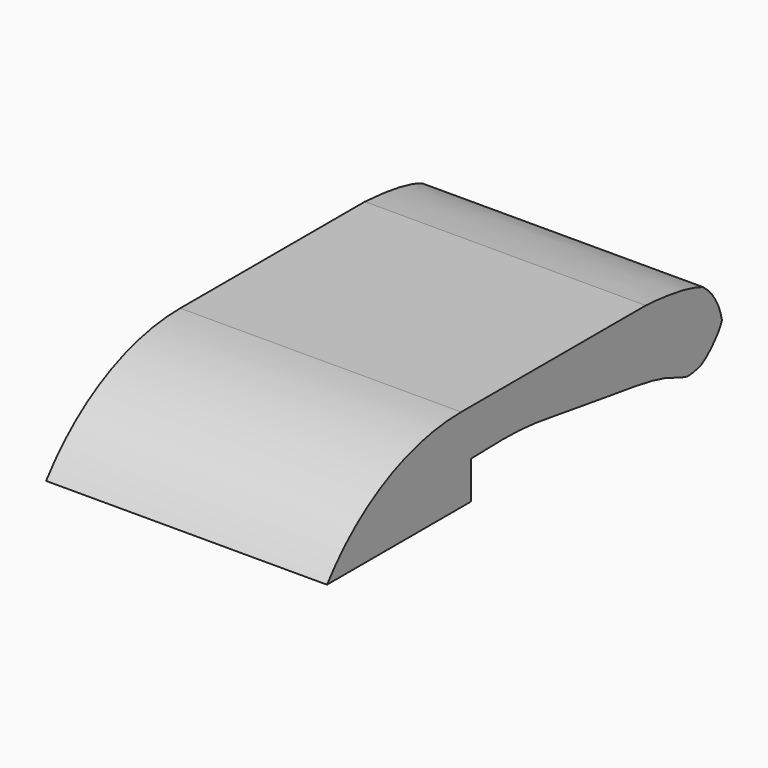
from build123d import *

# Parameters (mm, degrees)
F0_W        = 67
F0_H        = 20
F1_DEPTH    = 118
F3_T1_DEPTH = 267
F4_R        = 15
F5_T1_DEPTH = 122.9016994375
F6_DEPTH    = 67.001
F7_R        = 0.0241421356


# Not quite as in the source:
# - a fillet or chamfer that OpenCascade refuses, or shapes differently, is made with other operations: its cross-section is extruded or revolved along the edge and cut away or added


with BuildPart() as f1:
    # F0 (on Front) → F1 (new body)
    with BuildSketch(Plane.XZ):
        with Locations((6.337375957, -47.2683286667)):
            Rectangle(F0_W, F0_H)
    extrude(amount=F1_DEPTH)

    # F3: fillet of radius 50 on 1 edges, made by hand

    # F3_s2 → F3_t1 (cut)
    with BuildSketch(Plane.YZ.offset(-127.162624043)):
        with BuildLine():
            ThreePointArc((-78, -37.2683286667), (-100.360679775, -42.5469691167), (-118, -57.2683286667))
            Line((-118, -57.2683286667), (-118, -37.2683286667))
            Line((-118, -37.2683286667), (-78, -37.2683286667))
        make_face()
    extrude(amount=F3_T1_DEPTH, mode=Mode.SUBTRACT)

    # F4
    f4_edges = [f1.edges().sort_by_distance(p)[0] for p in [
        (6.337376, -78, -37.268329),
        (6.337376, 0, -37.268329),
    ]]
    fillet(f4_edges, radius=F4_R)

    # F5: fillet of radius 15 on 1 edges, made by hand

    # F5_s2 → F5_t1 (cut)
    with BuildSketch(Plane.YZ.offset(-55.1134737617)):
        with BuildLine():
            ThreePointArc((0, -52.2683286667), (-5.0566155305, -55.9613926043), (-11.1803398875, -57.2683286667))
            Line((-11.1803398875, -57.2683286667), (0, -57.2683286667))
            Line((0, -57.2683286667), (0, -52.2683286667))
        make_face()
    extrude(amount=F5_T1_DEPTH, mode=Mode.SUBTRACT)

    # F2 (on face) → F6 (cut, through all)
    with BuildSketch(Plane.YZ.offset(39.837375957)):
        with BuildLine():
            Line((-75, -48.2683286667), (-75, -57.2683286667))
            Line((-75, -57.2683286667), (-10.1939006259, -57.2683286667))
            add(Edge.make_bspline(
                [(-75, -48.2683286667), (-69.6300083872, -48.0932397516), (-59.1455400015, -47.7513929988), (-45.397034891, -50.3214203198), (-27.6071602735, -52.6118617406), (-16.9114345494, -54.5205994978), (-11.9954400696, -57.0260607697), (-10.1939006259, -57.2683286667)],
                knots=[0, 0, 0, 0, 0.1168750086, 0.2281888728, 0.353191241, 0.4546285253, 0.5170585623, 0.5170585623, 0.5170585623, 0.5170585623], degree=3))
        make_face()
        with BuildLine():
            add(Edge.make_bspline(
                [(-8.5831200704, -57.2683286667), (-6.3182593416, -56.9222504863), (-2.2304747887, -53.2529046852), (-0.154748351, -50.0842721126), (0, -48.2683286667)],
                knots=[0.5358591005, 0.5358591005, 0.5358591005, 0.5358591005, 0.6158678035, 0.6848581677, 0.6848581677, 0.6848581677, 0.6848581677], degree=3))
            Line((-8.5831200704, -57.2683286667), (0, -57.2683286667))
            Line((0, -57.2683286667), (0, -48.2683286667))
        make_face()
        with BuildLine():
            Line((0, -37.2683286667), (-22.9681972414, -37.2683286667))
            add(Edge.make_bspline(
                [(0, -47.2220127929), (-0.1541112697, -45.3649297857), (-3.0721745265, -39.2455424759), (-16.4826181453, -37.6339263761), (-22.9681972414, -37.2683286667)],
                knots=[0.69771165, 0.69771165, 0.69771165, 0.69771165, 0.7644699458, 0.8970561658, 0.8970561658, 0.8970561658, 0.8970561658], degree=3))
            Line((0, -47.2220127929), (0, -37.2683286667))
        make_face()
    extrude(amount=-F6_DEPTH, mode=Mode.SUBTRACT)

    # F7
    f7_edges = [f1.edges().sort_by_distance(p)[0] for p in [
        (6.337376, -0.250596, -49.53793),
        (-27.162624, -2.21712, -44.41989),
        (6.337376, -5.891526, -40.350456),
        (39.837376, -2.21712, -44.41989),
    ]]
    fillet(f7_edges, radius=F7_R)


solid = f1.part
